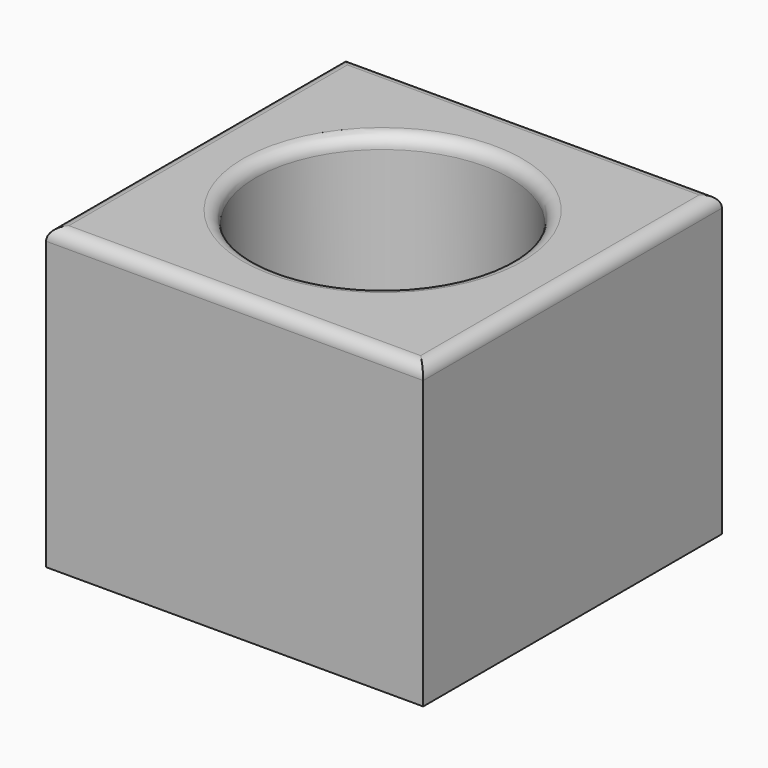
from build123d import *

# Parameters (mm, degrees)
F0_W     = 151.0536894202
F0_H     = 149.5463699102
F1_DEPTH = 60
F3_D     = 101.6
F2_R     = 50.8282360812
F4_DEPTH = 25.4
F8_R     = 5.08


# Not quite as in the source:
# - the program builds the solid bodies; features that only make, move or delete a surface that nothing else refers to are left out


with BuildPart() as f1:
    # F0 (on Top) → F1 (new body, symmetric)
    with BuildSketch(Plane.XY):
        with Locations((0.4253648221, 0.1466497779)):
            Rectangle(F0_W, F0_H)
    extrude(amount=F1_DEPTH, both=True)

    # F3 (through all)
    with Locations(Plane(origin=(0, 0, -60), x_dir=(1, 0, 0), z_dir=(0, 0, -1))):
        with Locations((0, 0)):
            Hole(F3_D / 2)

    # F2 (on face) → F4 (join)
    with BuildSketch(Plane(origin=(0, 0, -60), x_dir=(1, 0, 0), z_dir=(0, 0, -1))):
        Circle(F2_R)
    extrude(amount=-F4_DEPTH)

    # F8
    f8_edges = [f1.edges().sort_by_distance(p)[0] for p in [
        (-75.10148, 0.14665, 60),
        (0.425365, 74.919835, 60),
        (0.425365, -74.626535, 60),
        (75.95221, 0.14665, 60),
        (-50.8, 0, 60),
    ]]
    fillet(f8_edges, radius=F8_R)


solid = f1.part
